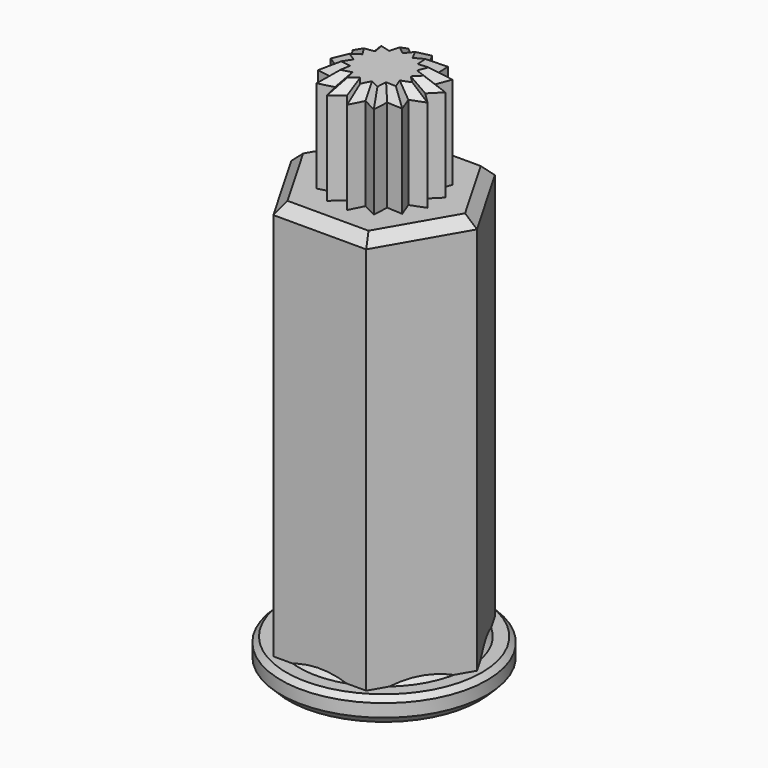
from build123d import *

# Parameters (mm, degrees)
F0_R      = 8
F1_DEPTH  = 2
F2_R      = 1
F2_R_2    = 1.6
F3_DEPTH  = 10
F4_R      = 6.2
F5_DEPTH  = 3
F7_DEPTH  = 25
F8_R      = 6
F8_R_2    = 1.8
F9_DEPTH  = 2
F10_SIZE  = 0.6
F11_SIZE  = 0.4
F13_DEPTH = 30
F15_DEPTH = 25
F17_DEPTH = 3
F18_SIZE  = 0.8
F20_DEPTH = 8
F21_SIZE  = 0.8


# Not quite as in the source:
# - a feature names something its author has since deleted; it is built from what else it names


with BuildPart() as f1:
    # F0 (on Top) → F1 (new body)
    with BuildSketch(Plane.XY):
        Circle(F0_R)
    extrude(amount=F1_DEPTH)

    # F2 (on face) → F3 (cut)
    with BuildSketch(Plane.XY.offset(2)):
        with Locations((11, 0)):
            Circle(F2_R)
        with Locations((0, 11)):
            Circle(F2_R)
        with Locations((-11, 0)):
            Circle(F2_R)
        with Locations((0, -11)):
            Circle(F2_R)
        with Locations((16, 0)):
            Circle(F2_R_2)
        with Locations((0, 16)):
            Circle(F2_R_2)
        with Locations((-16, 0)):
            Circle(F2_R_2)
        with Locations((0, -16)):
            Circle(F2_R_2)
        with BuildLine():
            ThreePointArc((8.909545443, 8.909545443), (6.6468037432, 8.909545443), (6.6468037432, 6.6468037432))
            Line((6.6468037432, 6.6468037432), (7.7781745931, 7.7781745931))
            Line((7.7781745931, 7.7781745931), (8.909545443, 8.909545443))
        make_face()
        with BuildLine():
            ThreePointArc((12.1018821522, 11.1018821522), (10.7191987199, 12.0257616848), (10.3947753711, 10.3947753711))
            ThreePointArc((10.3947753711, 10.3947753711), (11.4845655846, 10.1780026197), (12.1018821522, 11.1018821522))
        make_face()
        with BuildLine():
            Line((7.7781745931, 7.7781745931), (6.6468037432, 6.6468037432))
            ThreePointArc((6.6468037432, 6.6468037432), (8.3904680848, 6.299967341), (9.3781745931, 7.7781745931))
            ThreePointArc((9.3781745931, 7.7781745931), (9.2563818451, 8.3904680848), (8.909545443, 8.909545443))
            Line((8.909545443, 8.909545443), (7.7781745931, 7.7781745931))
        make_face()
        with Locations((-7.7781745931, 7.7781745931)):
            Circle(F2_R_2)
        with Locations((-11.1018821522, 11.1018821522)):
            Circle(F2_R)
        with Locations((-7.7781745931, -7.7781745931)):
            Circle(F2_R_2)
        with Locations((-11.1018821522, -11.1018821522)):
            Circle(F2_R)
        with Locations((7.7781745931, -7.7781745931)):
            Circle(F2_R_2)
        with Locations((11.1018821522, -11.1018821522)):
            Circle(F2_R)
    extrude(amount=-F3_DEPTH, mode=Mode.SUBTRACT)

    # F4 (on face) → F5 (join)
    with BuildSketch(Plane.XY.offset(2)):
        Circle(F4_R)
    extrude(amount=F5_DEPTH)

    # F6 (on face) → F7 (cut)
    with BuildSketch(Plane.XY.offset(5)):
        Polygon((3.2997422478, -0.4344193083), (2.8, 0), (3.2997422478, 0.4344193083), (2.7045923136, 0.7246933263), (3.0748702667, 1.273652967), (2.4248711306, 1.4), (2.6404509584, 2.0260892808), (1.9798989873, 1.9798989873), (2.0260892808, 2.6404509584), (1.4, 2.4248711306), (1.273652967, 3.0748702667), (0.7246933263, 2.7045923136), (0.4344193083, 3.2997422478), (0, 2.8), (-0.4344193083, 3.2997422478), (-0.7246933263, 2.7045923136), (-1.273652967, 3.0748702667), (-1.4, 2.4248711306), (-2.0260892808, 2.6404509584), (-1.9798989873, 1.9798989873), (-2.6404509584, 2.0260892808), (-2.4248711306, 1.4), (-3.0748702667, 1.273652967), (-2.7045923136, 0.7246933263), (-3.2997422478, 0.4344193083), (-2.8, 0), (-3.2997422478, -0.4344193083), (-2.7045923136, -0.7246933263), (-3.0748702667, -1.273652967), (-2.4248711306, -1.4), (-2.6404509584, -2.0260892808), (-1.9798989873, -1.9798989873), (-2.0260892808, -2.6404509584), (-1.4, -2.4248711306), (-1.273652967, -3.0748702667), (-0.7246933263, -2.7045923136), (-0.4344193083, -3.2997422478), (0, -2.8), (0.4344193083, -3.2997422478), (0.7246933263, -2.7045923136), (1.273652967, -3.0748702667), (1.4, -2.4248711306), (2.0260892808, -2.6404509584), (1.9798989873, -1.9798989873), (2.6404509584, -2.0260892808), (2.4248711306, -1.4), (3.0748702667, -1.273652967), (2.7045923136, -0.7246933263), align=None)
    extrude(amount=-F7_DEPTH, mode=Mode.SUBTRACT)

    # F8 (on Top) → F9 (join)
    with BuildSketch(Plane.XY):
        Circle(F8_R)
        Circle(F8_R_2, mode=Mode.SUBTRACT)
    extrude(amount=F9_DEPTH)

    # F10
    f10_edges = [f1.edges().sort_by_distance(p)[0] for p in [
        (-8, 0, 0),
        (-1.8, 0, 0),
    ]]
    chamfer(f10_edges, length=F10_SIZE)

    # F11
    f11_edges = [f1.edges().sort_by_distance(p)[0] for p in [
        (-6.2, 0, 5),
        (0.999173, -2.889731, 5),
        (1.336826, -2.749871, 5),
        (1.713045, -2.532661, 5),
        (2.002994, -2.310175, 5),
        (2.310175, -2.002994, 5),
        (2.532661, -1.713045, 5),
        (2.749871, -1.336826, 5),
        (2.889731, -0.999173, 5),
        (3.002167, -0.579556, 5),
        (3.049871, -0.21721, 5),
        (3.049871, 0.21721, 5),
        (3.002167, 0.579556, 5),
        (2.889731, 0.999173, 5),
        (2.749871, 1.336826, 5),
        (2.532661, 1.713045, 5),
        (2.310175, 2.002994, 5),
        (2.002994, 2.310175, 5),
        (1.713045, 2.532661, 5),
        (1.336826, 2.749871, 5),
        (0.999173, 2.889731, 5),
        (0.579556, 3.002167, 5),
        (0.21721, 3.049871, 5),
        (-0.21721, 3.049871, 5),
        (-0.579556, 3.002167, 5),
        (-0.999173, 2.889731, 5),
        (-1.336826, 2.749871, 5),
        (-1.713045, 2.532661, 5),
        (-2.002994, 2.310175, 5),
        (-2.310175, 2.002994, 5),
        (-2.532661, 1.713045, 5),
        (-2.749871, 1.336826, 5),
        (-2.889731, 0.999173, 5),
        (-3.002167, 0.579556, 5),
        (-3.049871, 0.21721, 5),
        (-3.049871, -0.21721, 5),
        (-3.002167, -0.579556, 5),
        (-2.889731, -0.999173, 5),
        (-2.749871, -1.336826, 5),
        (-2.532661, -1.713045, 5),
        (-2.310175, -2.002994, 5),
        (-2.002994, -2.310175, 5),
        (-1.713045, -2.532661, 5),
        (-1.336826, -2.749871, 5),
        (-0.999173, -2.889731, 5),
        (-0.579556, -3.002167, 5),
        (-0.21721, -3.049871, 5),
        (0.21721, -3.049871, 5),
        (0.579556, -3.002167, 5),
        (-8, 0, 2),
        (-6.2, 0, 2),
    ]]
    chamfer(f11_edges, length=F11_SIZE)


with BuildPart() as f13:
    # F12 (on Top) → F13 (new body)
    with BuildSketch(Plane.XY):
        Polygon((3.6084391824, 6.25), (-3.6084391824, 6.25), (-7.2168783649, 0), (-3.6084391824, -6.25), (3.6084391824, -6.25), (7.2168783649, 0), align=None)
    extrude(amount=F13_DEPTH)

    # F14 (on face) → F15 (cut)
    with BuildSketch(Plane(origin=(0, 0, 0), x_dir=(1, 0, 0), z_dir=(0, 0, -1))):
        Polygon((1.9629909152, 3.4), (-1.9629909152, 3.4), (-3.9259818305, 0), (-1.9629909152, -3.4), (1.9629909152, -3.4), (3.9259818305, 0), align=None)
    extrude(amount=-F15_DEPTH, mode=Mode.SUBTRACT)

    # F16 (on face) → F17 (join)
    with BuildSketch(Plane.XY.offset(30)):
        Polygon((3.6084391824, 6.25), (-3.6084391824, 6.25), (-7.2168783649, 0), (-3.6084391824, -6.25), (3.6084391824, -6.25), (7.2168783649, 0), align=None)
    extrude(amount=F17_DEPTH)

    # F18
    f18_edges = [f13.edges().sort_by_distance(p)[0] for p in [
        (5.412659, 3.125, 33),
        (0, 6.25, 33),
        (-5.412659, 3.125, 33),
        (-5.412659, -3.125, 33),
        (0, -6.25, 33),
        (5.412659, -3.125, 33),
        (0, 6.25, 0),
        (5.412659, 3.125, 0),
        (-5.412659, 3.125, 0),
        (5.412659, -3.125, 0),
        (-5.412659, -3.125, 0),
        (0, -6.25, 0),
        (2.944486, -1.7, 0),
        (2.944486, 1.7, 0),
        (0, 3.4, 0),
        (-2.944486, 1.7, 0),
        (-2.944486, -1.7, 0),
        (0, -3.4, 0),
    ]]
    chamfer(f18_edges, length=F18_SIZE)

    # F19 (on face) → F20 (join)
    with BuildSketch(Plane.XY.offset(33)):
        Polygon((4.0637839421, -0.8637839421), (3.2, 0), (4.0637839421, 0.8637839421), (2.9233454645, 1.3015572578), (3.3611187802, 2.4419957355), (2.1412179403, 2.3780634415), (2.0772856464, 3.5979642814), (0.988854382, 3.0433808521), (0.4342709528, 4.1318121165), (-0.3344910825, 3.1824700652), (-1.2838331338, 3.9512321004), (-1.6, 2.7712812921), (-2.7799508083, 3.0874481583), (-2.588854382, 1.8809128073), (-3.795389733, 1.689816381), (-3.1300723223, 0.6653174106), (-4.1545712928, 0), (-3.1300723223, -0.6653174106), (-3.795389733, -1.689816381), (-2.588854382, -1.8809128073), (-2.7799508083, -3.0874481583), (-1.6, -2.7712812921), (-1.2838331338, -3.9512321004), (-0.3344910825, -3.1824700652), (0.4342709528, -4.1318121165), (0.988854382, -3.0433808521), (2.0772856464, -3.5979642814), (2.1412179403, -2.3780634415), (3.3611187802, -2.4419957355), (2.9233454645, -1.3015572578), align=None)
    extrude(amount=F20_DEPTH)

    # F21
    f21_edges = [f13.edges().sort_by_distance(p)[0] for p in [
        (3.631892, -0.431892, 41),
        (3.631892, 0.431892, 41),
        (3.493565, 1.082671, 41),
        (3.142232, 1.871776, 41),
        (2.751168, 2.41003, 41),
        (2.109252, 2.988014, 41),
        (1.53307, 3.320673, 41),
        (0.711563, 3.587596, 41),
        (0.04989, 3.657141, 41),
        (-0.809162, 3.566851, 41),
        (-1.441917, 3.361257, 41),
        (-2.189975, 2.929365, 41),
        (-2.684403, 2.48418, 41),
        (-3.192122, 1.785365, 41),
        (-3.462731, 1.177567, 41),
        (-3.642322, 0.332659, 41),
        (-3.642322, -0.332659, 41),
        (-3.462731, -1.177567, 41),
        (-3.192122, -1.785365, 41),
        (-2.684403, -2.48418, 41),
        (-2.189975, -2.929365, 41),
        (-1.441917, -3.361257, 41),
        (-0.809162, -3.566851, 41),
        (0.04989, -3.657141, 41),
        (0.711563, -3.587596, 41),
        (1.53307, -3.320673, 41),
        (2.109252, -2.988014, 41),
        (2.751168, -2.41003, 41),
        (3.142232, -1.871776, 41),
        (3.493565, -1.082671, 41),
    ]]
    chamfer(f21_edges, length=F21_SIZE)


solid = Compound([f1.part, f13.part])
